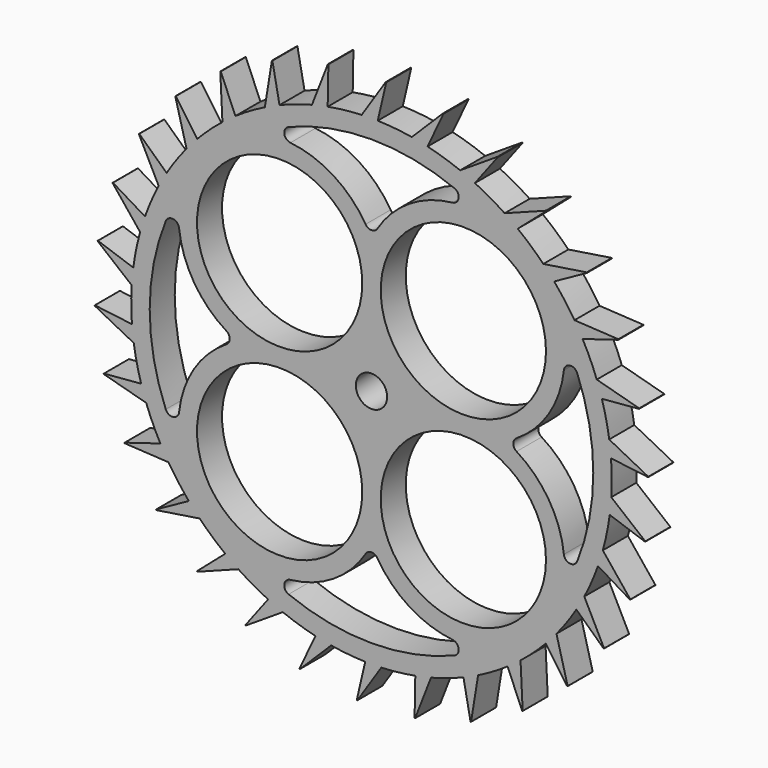
from build123d import *

# Parameters (mm, degrees)
F0_R     = 21.120769
F1_DEPTH = 8
F3_D     = 8


# Not quite as in the source:
# - ends of sketch curves that miss each other by under 0.0002 mm in the source are joined


with BuildPart() as f1:
    # F0 (on Front) → F1 (new body)
    with BuildSketch(Plane.XZ):
        with BuildLine():
            Line((-44.555484, 42.271698), (-50.011201, 50.086009))
            ThreePointArc((-50.011201, 50.086009), (-50.1057089701, 50.1092715418), (-50.1411099411, 50.0186100213))
            Line((-50.1411099411, 50.0186100213), (-47.284702, 39.194955))
            ThreePointArc((-47.284702, 39.194955), (-49.9543386998, 35.7302618175), (-52.3706196786, 32.0843538031))
            Line((-52.3706196786, 32.0843538031), (-59.331803, 38.593596))
            ThreePointArc((-59.331803, 38.593596), (-59.4290825445, 38.5967008994), (-59.4448600075, 38.5006599953))
            Line((-59.4448600075, 38.5006599953), (-54.400507, 28.507409))
            ThreePointArc((-54.400507, 28.507409), (-56.2914557492, 24.5633787196), (-57.8969084003, 20.4947691417))
            Line((-57.8969084003, 20.4947691417), (-66.059321, 25.414458))
            ThreePointArc((-66.059321, 25.414458), (-66.1551196477, 25.3972694202), (-66.1505846562, 25.3000473311))
            Line((-66.1505846562, 25.3000473311), (-59.138749, 16.573952))
            ThreePointArc((-59.138749, 16.573952), (-60.1683660284, 12.3229580038), (-60.8928241631, 8.0094650215))
            Line((-60.8928241631, 8.0094650215), (-69.899729, 11.124586))
            ThreePointArc((-69.899729, 11.124586), (-69.9898609706, 11.0878555231), (-69.9652112757, 10.9937005924))
            Line((-69.9652112757, 10.9937005924), (-61.292344, 3.916134))
            ThreePointArc((-61.292344, 3.916134), (-61.4156299049, -0.4560349502), (-61.2274312734, -4.8258910215))
            Line((-61.2274312734, -4.8258910215), (-70.685183, -3.651484))
            ThreePointArc((-70.685183, -3.651484), (-70.7657094788, -3.7061505191), (-70.7220221527, -3.7931233764))
            Line((-70.7220221527, -3.7931233764), (-60.76717, -8.912837))
            ThreePointArc((-60.76717, -8.912837), (-59.9787361929, -13.2150962612), (-58.8861059823, -17.4503319948))
            Line((-58.8861059823, -17.4503319948), (-68.381356, -18.267966))
            ThreePointArc((-68.381356, -18.267966), (-68.4487562267, -18.3381805548), (-68.3879419529, -18.4141697352))
            Line((-68.3879419529, -18.4141697352), (-57.586178, -21.352275))
            ThreePointArc((-57.586178, -21.352275), (-55.92048391, -25.3965951213), (-53.971175293, -29.3121101591))
            Line((-53.971175293, -29.3121101591), (-63.088936, -32.086051))
            ThreePointArc((-63.088936, -32.086051), (-63.1402645105, -32.1687442744), (-63.0649800148, -32.2304285583))
            Line((-63.0649800148, -32.2304285583), (-51.888394, -32.858517))
            ThreePointArc((-51.888394, -32.858517), (-49.4182379701, -36.4681411703), (-46.6974454013, -39.8928083428))
            Line((-46.6974454013, -39.8928083428), (-55.039226, -44.501821))
            ThreePointArc((-55.039226, -44.501821), (-55.0722405937, -44.5933785635), (-54.9857761498, -44.6380623958))
            Line((-54.9857761498, -44.6380623958), (-43.922838, -42.928683))
            ThreePointArc((-43.922838, -42.928683), (-40.7561779448, -45.9458542615), (-37.3828127854, -48.7299997203))
            Line((-37.3828127854, -48.7299997203), (-44.584038, -54.972648))
            ThreePointArc((-44.584038, -54.972648), (-44.5972948673, -55.0690686912), (-44.5034301957, -55.0947995974))
            Line((-44.5034301957, -55.0947995974), (-34.037644, -51.12266))
            ThreePointArc((-34.037644, -51.12266), (-30.3128775663, -53.4155128978), (-26.434372048, -55.4374561007))
            Line((-26.434372048, -55.4374561007), (-32.180314, -63.040906))
            ThreePointArc((-32.180314, -63.040906), (-32.173233533, -63.1379765095), (-32.0760699992, -63.143629001))
            Line((-32.0760699992, -63.143629001), (-22.664841, -57.082331))
            ThreePointArc((-22.664841, -57.082331), (-18.5447587661, -58.5506574412), (-14.3306221704, -59.7220297101))
            Line((-14.3306221704, -59.7220297101), (-18.370155, -68.353975))
            ThreePointArc((-18.370155, -68.353975), (-18.3430479667, -68.4474516438), (-18.2468324399, -68.4327786298))
            Line((-18.2468324399, -68.4327786298), (-10.301476, -60.54723))
            ThreePointArc((-10.301476, -60.54723), (-5.9661449458, -61.126857264), (-1.6005549993, -61.3964639713))
            Line((-1.6005549993, -61.3964639713), (-3.757133, -70.679646))
            ThreePointArc((-3.757133, -70.679646), (-3.7111832792, -70.7654451744), (-3.6201204676, -70.7310887505))
            Line((-3.6201204676, -70.7310887505), (2.512113, -61.365925))
            ThreePointArc((2.512113, -61.365925), (6.8732176273, -61.0315200854), (11.1994630242, -60.3875781304))
            Line((11.1994630242, -60.3875781304), (11.020094, -69.916278))
            ThreePointArc((11.020094, -69.916278), (11.0828788815, -69.9906481657), (11.1648084181, -69.9381098323))
            Line((11.1648084181, -69.9381098323), (15.215911, -59.502635))
            ThreePointArc((15.215911, -59.502635), (19.4121879494, -58.2688126145), (23.5100111832, -56.7394654421))
            Line((23.5100111832, -56.7394654421), (25.315691, -66.097233))
            ThreePointArc((25.315691, -66.097233), (25.3925651998, -66.1569244795), (25.4617809719, -66.088499998))
            Line((25.4617809719, -66.088499998), (27.2547, -55.038794))
            ThreePointArc((27.2547, -55.038794), (31.1027524032, -52.9594784475), (34.7930594527, -50.6115656585))
            Line((34.7930594527, -50.6115656585), (38.504869, -59.389422))
            ThreePointArc((38.504869, -59.389422), (38.5924747473, -59.431825865), (38.6459519714, -59.350506004))
            Line((38.6459519714, -59.350506004), (38.102328, -48.169493))
            ThreePointArc((38.102328, -48.169493), (41.4339776661, -45.3355606478), (44.5554842525, -42.2716972396))
            Line((44.5554842525, -42.2716972396), (50.011201, -50.086008))
            ThreePointArc((50.011201, -50.086008), (50.1057081263, -50.1092714607), (50.1411087369, -50.0186094578))
            Line((50.1411087369, -50.0186094578), (47.284702, -39.194955))
            ThreePointArc((47.284702, -39.194955), (49.9543387959, -35.7302616832), (52.3706198512, -32.0843535215))
            Line((52.3706198512, -32.0843535215), (59.331803, -38.593595))
            ThreePointArc((59.331803, -38.593595), (59.4290813586, -38.5967010522), (59.4448592871, -38.5006604441))
            Line((59.4448592871, -38.5006604441), (54.400507, -28.507409))
            ThreePointArc((54.400507, -28.507409), (56.2914557492, -24.5633787196), (57.8969084003, -20.4947691417))
            Line((57.8969084003, -20.4947691417), (66.05932, -25.414457))
            ThreePointArc((66.05932, -25.414457), (66.1551184867, -25.397269622), (66.1505836562, -25.3000473311))
            Line((66.1505836562, -25.3000473311), (59.138749, -16.573952))
            ThreePointArc((59.138749, -16.573952), (60.1683660284, -12.3229580038), (60.8928241631, -8.0094650215))
            Line((60.8928241631, -8.0094650215), (69.899728, -11.124585))
            ThreePointArc((69.899728, -11.124585), (69.9898598376, -11.0878557891), (69.9652104976, -10.9937007425))
            Line((69.9652104976, -10.9937007425), (61.292344, -3.916134))
            ThreePointArc((61.292344, -3.916134), (61.4156299049, 0.4560349502), (61.2274312734, 4.8258910215))
            Line((61.2274312734, 4.8258910215), (70.685183, 3.651484))
            ThreePointArc((70.685183, 3.651484), (70.7657085343, 3.7061507328), (70.7220216631, 3.7931231694))
            Line((70.7220216631, 3.7931231694), (60.767169, 8.912838))
            ThreePointArc((60.767169, 8.912838), (59.9787360402, 13.2150969539), (58.8861059016, 17.4503322672))
            Line((58.8861059016, 17.4503322672), (68.381356, 18.267967))
            ThreePointArc((68.381356, 18.267967), (68.4487562508, 18.3381810894), (68.3879409836, 18.4141699075))
            Line((68.3879409836, 18.4141699075), (57.586177, 21.352276))
            ThreePointArc((57.586177, 21.352276), (55.9204834626, 25.3965961065), (53.9711748736, 29.3121109313))
            Line((53.9711748736, 29.3121109313), (63.088935, 32.086051))
            ThreePointArc((63.088935, 32.086051), (63.140264507, 32.1687442955), (63.0649790159, 32.2304285248))
            Line((63.0649790159, 32.2304285248), (51.888394, 32.858517))
            ThreePointArc((51.888394, 32.858517), (49.4182377444, 36.4681414762), (46.6974449074, 39.8928089209))
            Line((46.6974449074, 39.8928089209), (55.039226, 44.501821))
            ThreePointArc((55.039226, 44.501821), (55.0722394782, 44.5933798578), (54.9857749162, 44.6380633379))
            Line((54.9857749162, 44.6380633379), (43.922838, 42.928683))
            ThreePointArc((43.922838, 42.928683), (40.756177648, 45.9458545248), (37.3828121559, 48.7300002032))
            Line((37.3828121559, 48.7300002032), (44.584038, 54.972648))
            ThreePointArc((44.584038, 54.972648), (44.5972946796, 55.0690699756), (44.5034289936, 55.0948000131))
            Line((44.5034289936, 55.0948000131), (34.037643, 51.12266))
            ThreePointArc((34.037643, 51.12266), (30.3128768118, 53.415513326), (26.4343712333, 55.4374564892))
            Line((26.4343712333, 55.4374564892), (32.180313, 63.040907))
            ThreePointArc((32.180313, 63.040907), (32.1732334667, 63.1379775748), (32.0760693769, 63.1436295162))
            Line((32.0760693769, 63.1436295162), (22.664841, 57.082331))
            ThreePointArc((22.664841, 57.082331), (18.5447586549, 58.5506574764), (14.3306219435, 59.7220297646))
            Line((14.3306219435, 59.7220297646), (18.370155, 68.353975))
            ThreePointArc((18.370155, 68.353975), (18.343047441, 68.4474523407), (18.2468318545, 68.4327801225))
            Line((18.2468318545, 68.4327801225), (10.301475, 60.547231))
            ThreePointArc((10.301475, 60.547231), (5.9661443718, 61.12685732), (1.6005549993, 61.3964639713))
            Line((1.6005549993, 61.3964639713), (3.757132, 70.679647))
            ThreePointArc((3.757132, 70.679647), (3.7111820436, 70.7654452629), (3.6201196892, 70.7310891658))
            Line((3.6201196892, 70.7310891658), (-2.512114, 61.365926))
            ThreePointArc((-2.512114, 61.365926), (-6.873218592, 61.0315199768), (-11.1994639909, 60.3875779511))
            Line((-11.1994639909, 60.3875779511), (-11.020095, 69.916279))
            ThreePointArc((-11.020095, 69.916279), (-11.0828793473, 69.9906492359), (-11.1648086842, 69.938109909))
            Line((-11.1648086842, 69.938109909), (-15.215911, 59.502635))
            ThreePointArc((-15.215911, 59.502635), (-19.4121883876, 58.2688124685), (-23.5100120366, 56.7394650884))
            Line((-23.5100120366, 56.7394650884), (-25.315691, 66.097234))
            ThreePointArc((-25.315691, 66.097234), (-25.3925661052, 66.1569254851), (-25.4617819719, 66.088500998))
            Line((-25.4617819719, 66.088500998), (-27.254701, 55.038794))
            ThreePointArc((-27.254701, 55.038794), (-31.1027529006, 52.9594781554), (-34.7930596649, 50.6115655126))
            Line((-34.7930596649, 50.6115655126), (-38.50487, 59.389422))
            ThreePointArc((-38.50487, 59.389422), (-38.5924749021, 59.4318268223), (-38.6459518539, 59.3505061595))
            Line((-38.6459518539, 59.3505061595), (-38.102329, 48.169494))
            ThreePointArc((-38.102329, 48.169494), (-41.4339774589, 45.3355608372), (-44.555484, 42.271698))
        make_face()
        with Locations((-23.482974, -23.482973)):
            Circle(F0_R, mode=Mode.SUBTRACT)
        with BuildLine():
            ThreePointArc((-21.1888832768, -52.5843866869), (-22.2815668488, -50.6975895271), (-20.7163770495, -49.1796495405))
            ThreePointArc((-20.7163770495, -49.1796495405), (-9.7124443099, -45.3540895217), (-1.5064622486, -37.0846698461))
            ThreePointArc((-1.5064622486, -37.0846698461), (-2.631e-07, -36.245395), (1.5064616123, -37.084669621))
            ThreePointArc((1.5064616123, -37.084669621), (9.7124437306, -45.3540897866), (20.7163770754, -49.1796492995))
            ThreePointArc((20.7163770754, -49.1796492995), (22.2815658534, -50.6975895601), (21.1888831371, -52.5843863402))
            ThreePointArc((21.1888831371, -52.5843863402), (0, -56.692913), (-21.1888832768, -52.5843866869))
        make_face(mode=Mode.SUBTRACT)
        with Locations((23.482973, -23.482973)):
            Circle(F0_R, mode=Mode.SUBTRACT)
        with BuildLine():
            ThreePointArc((-52.5843866869, 21.1888832768), (-50.6975895271, 22.2815668488), (-49.1796495405, 20.7163770495))
            ThreePointArc((-49.1796495405, 20.7163770495), (-45.3540904932, 9.7124442646), (-37.0846708461, 1.5064622486))
            ThreePointArc((-37.0846708461, 1.5064622486), (-36.245395, 2.631e-07), (-37.0846703441, -1.5064620598))
            ThreePointArc((-37.0846703441, -1.5064620598), (-45.354090758, -9.7124436853), (-49.1796502881, -20.716376969))
            ThreePointArc((-49.1796502881, -20.716376969), (-50.6975895601, -22.2815658534), (-52.5843863402, -21.1888831371))
            ThreePointArc((-52.5843863402, -21.1888831371), (-56.692913, 0), (-52.5843866869, 21.1888832768))
        make_face(mode=Mode.SUBTRACT)
        with Locations((-23.482974, 23.482974)):
            Circle(F0_R, mode=Mode.SUBTRACT)
        with Locations((23.482973, 23.482974)):
            Circle(F0_R, mode=Mode.SUBTRACT)
        with BuildLine():
            ThreePointArc((52.5843863402, -21.1888831371), (50.6975895601, -22.2815658534), (49.1796496469, -20.716377038))
            ThreePointArc((49.1796496469, -20.716377038), (45.3540897866, -9.7124437306), (37.0846698461, -1.5064612486))
            ThreePointArc((37.0846698461, -1.5064612486), (36.245395, 2.631e-07), (37.0846700685, 1.5064618893))
            ThreePointArc((37.0846700685, 1.5064618893), (45.3540895217, 9.7124443099), (49.1796491931, 20.7163770869))
            ThreePointArc((49.1796491931, 20.7163770869), (50.6975895271, 22.2815668488), (52.5843866869, 21.1888832768))
            ThreePointArc((52.5843866869, 21.1888832768), (56.692913, 0), (52.5843863402, -21.1888831371))
        make_face(mode=Mode.SUBTRACT)
        with BuildLine():
            ThreePointArc((21.1888831371, 52.5843863402), (22.2815658534, 50.6975895601), (20.716377038, 49.1796496469))
            ThreePointArc((20.716377038, 49.1796496469), (9.7124436853, 45.354090758), (1.5064612486, 37.0846708461))
            ThreePointArc((1.5064612486, 37.0846708461), (-2.631e-07, 36.245395), (-1.5064623368, 37.0846707916))
            ThreePointArc((-1.5064623368, 37.0846707916), (-9.7124442646, 45.3540904932), (-20.7163769804, 49.1796501816))
            ThreePointArc((-20.7163769804, 49.1796501816), (-22.2815668488, 50.6975895271), (-21.1888832768, 52.5843866869))
            ThreePointArc((-21.1888832768, 52.5843866869), (0, 56.692913), (21.1888831371, 52.5843863402))
        make_face(mode=Mode.SUBTRACT)
    extrude(amount=F1_DEPTH)

    # F3 (through all)
    with Locations(Plane.XZ.offset(8)):
        with Locations((0, 0)):
            Hole(F3_D / 2)


solid = f1.part
